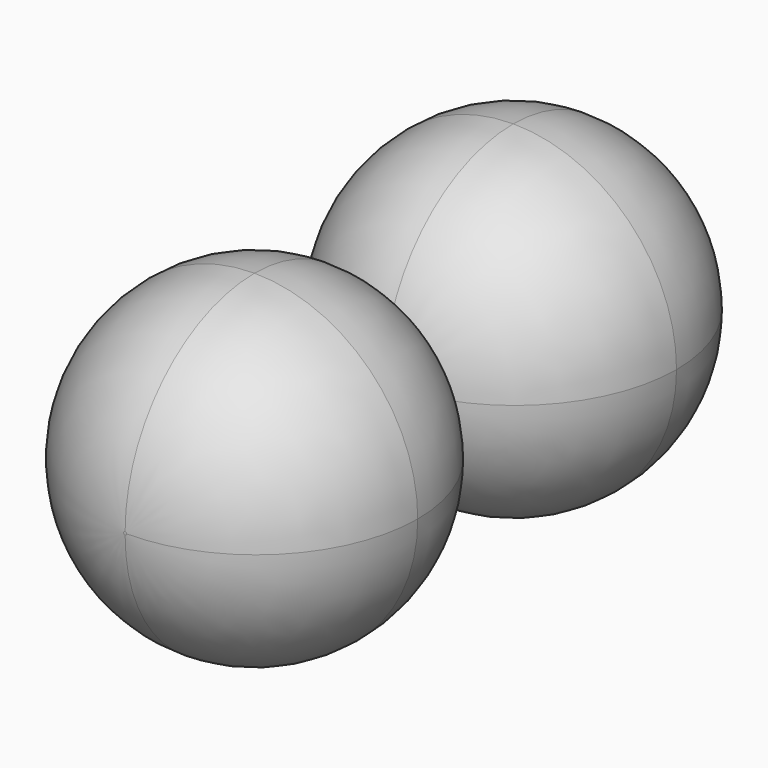
from build123d import *

# Parameters (mm, degrees)
F1_DEPTH = 76.2
F2_R     = 38.09999


# Not quite as in the source:
# - a fillet or chamfer is up to 0.001 mm smaller than in the source, because OpenCascade refuses the exact size


with BuildPart() as f1:
    # F0 (on Front) → F1 (new body)
    with BuildSketch(Plane.XZ):
        with BuildLine():
            ThreePointArc((0, -38.4565959736), (27.1929197943, -27.1929197943), (38.4565959736, 0))
            ThreePointArc((38.4565959736, 0), (27.1929197943, 27.1929197943), (0, 38.4565959736))
            Line((0, 38.4565959736), (0, -38.4565959736))
        make_face()
        with BuildLine():
            Line((0, -38.4565959736), (0, 38.4565959736))
            ThreePointArc((0, 38.4565959736), (-38.4565959736, 0), (0, -38.4565959736))
        make_face()
    extrude(amount=F1_DEPTH)

    # F2 (radius 38.1 in the source; OpenCascade refuses exactly that, so slightly less here)
    f2_edges = [f1.edges().sort_by_distance(p)[0] for p in [
        (38.456596, -38.1, 0),
        (-38.456596, 0, 0),
        (-38.456596, -76.2, 0),
    ]]
    fillet(f2_edges, radius=F2_R)

    # F3: F1 across plane


with BuildPart() as f1_1:
    add(f1.part)
    add(f1.part.mirror(Plane.XZ))


solid = f1_1.part
